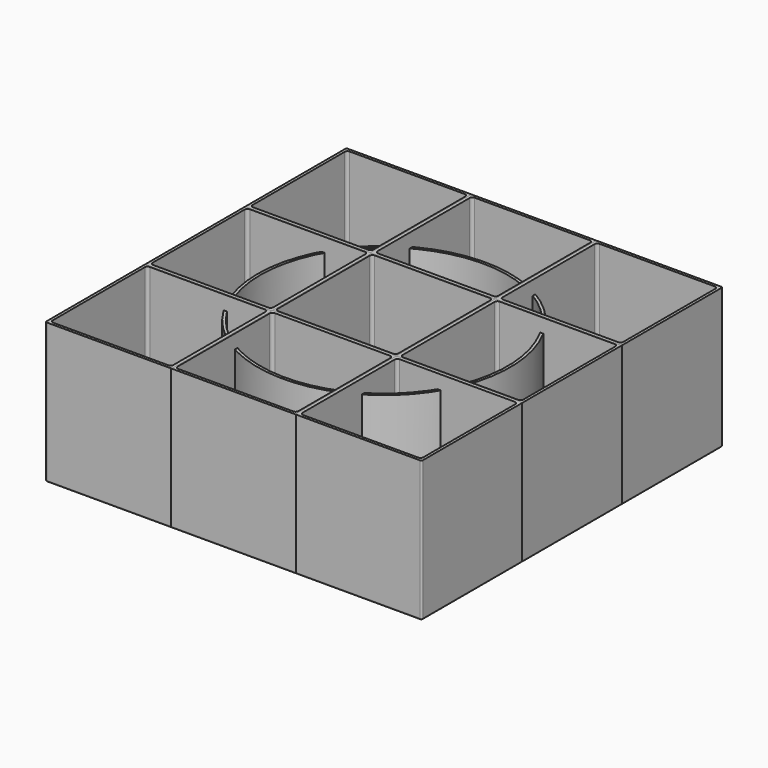
from build123d import *

# Parameters (mm, degrees)
F2_W         = 45
F2_H         = 45
F3_DEPTH     = 50
F4_T         = -1
F5_R         = 0.5
F6_R         = 0.5
F7_R         = 0.5
F8_T1_DEPTH  = 49
F8_T4_ANGLE  = 90
F8_T6_ANGLE  = 90
F8_T8_ANGLE  = 90
F8_T10_ANGLE = 90


# Not quite as in the source:
# - a fillet or chamfer that OpenCascade refuses, or shapes differently, is made with other operations: its cross-section is extruded or revolved along the edge and cut away or added


with BuildPart() as f1:
    # F0 (on Front) → F1 (revolve)
    with BuildSketch(Plane.XZ):
        Polygon((-45, 0), (0, 0), (0, 1), (-44, 1), (-44, 45), (-45, 45), align=None)
    revolve(axis=Axis((0, 0, 23), (0, 0, -1)))


with BuildPart() as f3:
    # F2 (on Top) → F3 (new body)
    with BuildSketch(Plane.XY):
        Rectangle(F2_W, F2_H)
    extrude(amount=F3_DEPTH)

    # F4
    f4_openings = [f3.faces().sort_by_distance(p)[0] for p in [
        (0, 0, 50),
    ]]
    offset(amount=F4_T, openings=f4_openings)

    # F5
    f5_edges = [f3.edges().sort_by_distance(p)[0] for p in [
        (22.5, 22.5, 25),
        (-22.5, 22.5, 25),
        (-22.5, -22.5, 25),
        (22.5, -22.5, 25),
    ]]
    fillet(f5_edges, radius=F5_R)

    # F6
    f6_edges = [f3.edges().sort_by_distance(p)[0] for p in [
        (22.5, 0, 0),
        (22.353553, -22.353553, 0),
        (22.353553, 22.353553, 0),
        (0, -22.5, 0),
        (0, 22.5, 0),
        (-22.353553, -22.353553, 0),
        (-22.353553, 22.353553, 0),
        (-22.5, 0, 0),
    ]]
    fillet(f6_edges, radius=F6_R)

    # F7
    f7_edges = [f3.edges().sort_by_distance(p)[0] for p in [
        (21.5, 0, 1),
        (0, 21.5, 1),
        (-21.5, 0, 1),
        (0, -21.5, 1),
    ]]
    fillet(f7_edges, radius=F7_R)

    # F8: fillet of radius 1 on 4 edges, made by hand

    # F8_s2 → F8_t1 (join)
    with BuildSketch(Plane.XY.offset(1)):
        with BuildLine():
            ThreePointArc((-20.5, 21.5), (-21.2071067812, 21.2071067812), (-21.5, 20.5))
            Line((-21.5, 20.5), (-21.5, 21.5))
            Line((-21.5, 21.5), (-20.5, 21.5))
        make_face()
        with BuildLine():
            ThreePointArc((-20.5, -21.5), (-21.2071067812, -21.2071067812), (-21.5, -20.5))
            Line((-21.5, -20.5), (-21.5, -21.5))
            Line((-21.5, -21.5), (-20.5, -21.5))
        make_face()
        with BuildLine():
            ThreePointArc((21.5, 20.5), (21.2071067812, 21.2071067812), (20.5, 21.5))
            Line((20.5, 21.5), (21.5, 21.5))
            Line((21.5, 21.5), (21.5, 20.5))
        make_face()
        with BuildLine():
            ThreePointArc((21.5, -20.5), (21.2071067812, -21.2071067812), (20.5, -21.5))
            Line((20.5, -21.5), (21.5, -21.5))
            Line((21.5, -21.5), (21.5, -20.5))
        make_face()
    extrude(amount=F8_T1_DEPTH)

    # F8_s3 → F8_t4 (revolve)
    with BuildSketch(Plane.XZ.offset(20.5)):
        with BuildLine():
            ThreePointArc((21, 1), (21.3535533906, 1.1464466094), (21.5, 1.5))
            Line((21.5, 1.5), (21.5, 1))
            Line((21.5, 1), (21, 1))
        make_face()
    revolve(axis=Axis((20.5, -20.5, 1), (0, 0, -1)), revolution_arc=F8_T4_ANGLE)

    # F8_s5 → F8_t6 (revolve)
    with BuildSketch(Plane.YZ.offset(20.5)):
        with BuildLine():
            ThreePointArc((21, 1), (21.3535533906, 1.1464466094), (21.5, 1.5))
            Line((21.5, 1.5), (21.5, 1))
            Line((21.5, 1), (21, 1))
        make_face()
    revolve(axis=Axis((20.5, 20.5, 1), (0, 0, -1)), revolution_arc=F8_T6_ANGLE)

    # F8_s7 → F8_t8 (revolve)
    with BuildSketch(Plane.YZ.offset(-20.5)):
        with BuildLine():
            ThreePointArc((-21, 1), (-21.3535533906, 1.1464466094), (-21.5, 1.5))
            Line((-21.5, 1.5), (-21.5, 1))
            Line((-21.5, 1), (-21, 1))
        make_face()
    revolve(axis=Axis((-20.5, -20.5, 1), (0, 0, -1)), revolution_arc=F8_T8_ANGLE)

    # F8_s9 → F8_t10 (revolve)
    with BuildSketch(Plane.XZ.offset(-20.5)):
        with BuildLine():
            ThreePointArc((-21, 1), (-21.3535533906, 1.1464466094), (-21.5, 1.5))
            Line((-21.5, 1.5), (-21.5, 1))
            Line((-21.5, 1), (-21, 1))
        make_face()
    revolve(axis=Axis((-20.5, 20.5, 1), (0, 0, -1)), revolution_arc=F8_T10_ANGLE)


with BuildPart() as f9_1:
    # F9: copy of F3
    add(f3.part.moved(Location((0, -44.5, 0))))


with BuildPart() as f10_1:
    # F10: copy of F9_1
    add(f9_1.part.moved(Location((-44.5, 0, 0))))


with BuildPart() as f11_1:
    # F11: copy of F3
    add(f3.part.moved(Location((-44.5, 0, 0))))


with BuildPart() as f12_1:
    # F12: copy of F11_1
    add(f11_1.part.moved(Location((0, 44.5, 0))))


with BuildPart() as f13_1:
    # F13: copy of F3
    add(f3.part.moved(Location((0, 44.5, 0))))


with BuildPart() as f14_1:
    # F14: copy of F3
    add(f3.part.moved(Location((44.5, 0, 0))))


with BuildPart() as f15_1:
    # F15: copy of F9_1
    add(f9_1.part.moved(Location((44.5, 0, 0))))


with BuildPart() as f16_1:
    # F16: copy of F13_1
    add(f13_1.part.moved(Location((44.5, 0, 0))))


solid = Compound([f1.part, f3.part, f9_1.part, f10_1.part, f11_1.part, f12_1.part, f13_1.part, f14_1.part, f15_1.part, f16_1.part])
